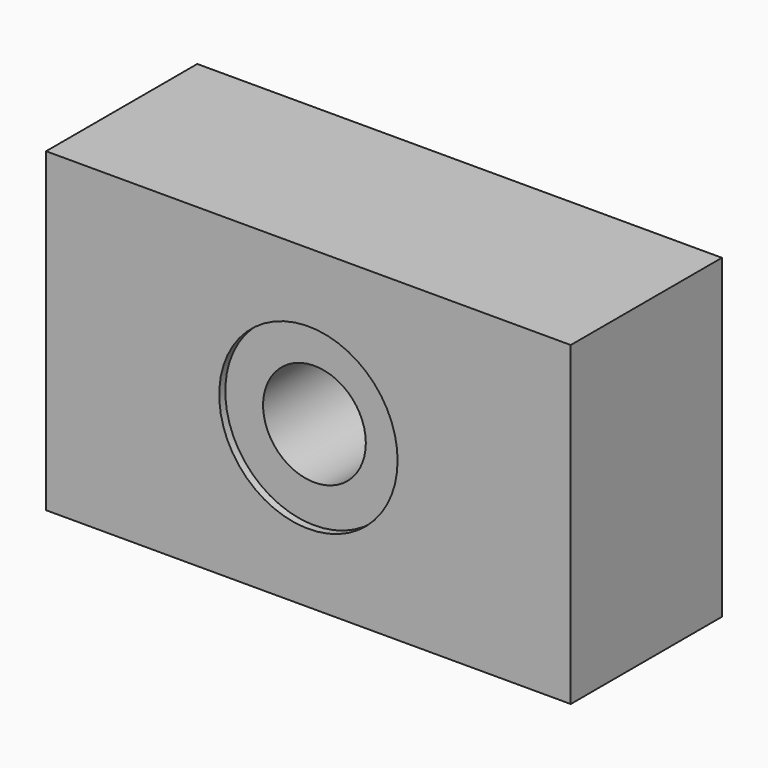
from build123d import *

# Parameters (mm, degrees)
F0_R     = 11.9868187185
F0_R_2   = 6.9041541384
F1_DEPTH = 24.384
F0_W     = 70.5220922828
F0_H     = 42.4831844866
F2_DEPTH = 25.4


# Not quite as in the source:
# - the program builds the solid bodies; features that only make, move or delete a surface that nothing else refers to are left out


with BuildPart() as f1:
    # F0 (on Front) → F1 (new body)
    with BuildSketch(Plane.XZ):
        Circle(F0_R)
        Circle(F0_R_2, mode=Mode.SUBTRACT)
    extrude(amount=F1_DEPTH)

    # F0 (on Front) → F2 (join)
    with BuildSketch(Plane.XZ):
        Rectangle(F0_W, F0_H)
        Circle(F0_R, mode=Mode.SUBTRACT)
    extrude(amount=F2_DEPTH)


solid = f1.part
